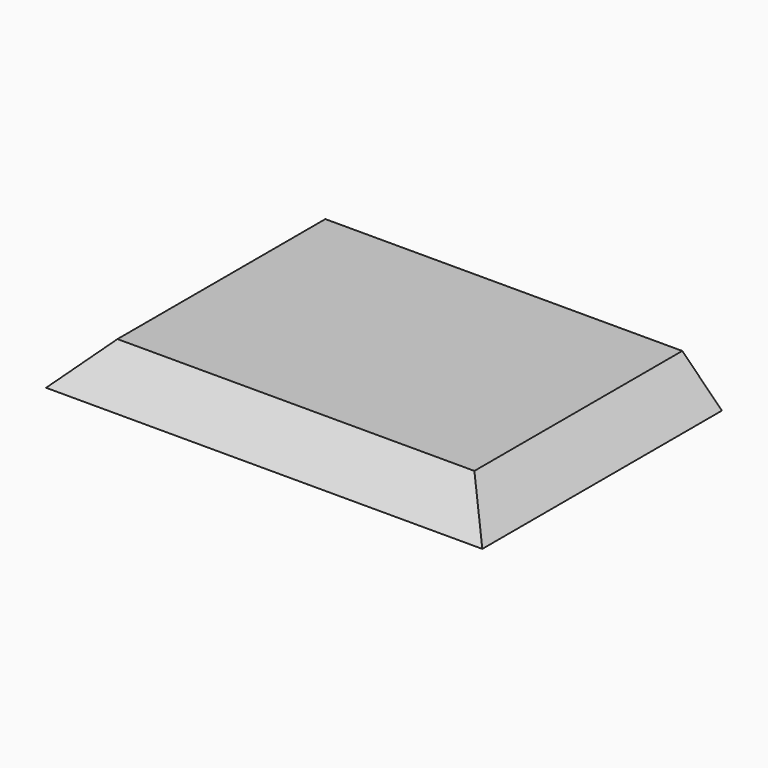
from build123d import *

# Parameters (mm, degrees)
F0_W     = 55
F0_H     = 37.76
F1_DEPTH = 5
F2_SIZE  = 4.99999


# Not quite as in the source:
# - a fillet or chamfer is up to 0.001 mm smaller than in the source, because OpenCascade refuses the exact size


with BuildPart() as f1:
    # F0 (on Top) → F1 (new body)
    with BuildSketch(Plane.XY):
        with Locations((0, -33.62)):
            Rectangle(F0_W, F0_H)
    extrude(amount=F1_DEPTH)

    # F2 (size 5 in the source; OpenCascade refuses exactly that, so slightly less here)
    f2_edges = [f1.edges().sort_by_distance(p)[0] for p in [
        (-27.5, -33.62, 5),
        (27.5, -33.62, 5),
        (0, -52.5, 5),
    ]]
    chamfer(f2_edges, length=F2_SIZE)


solid = f1.part
